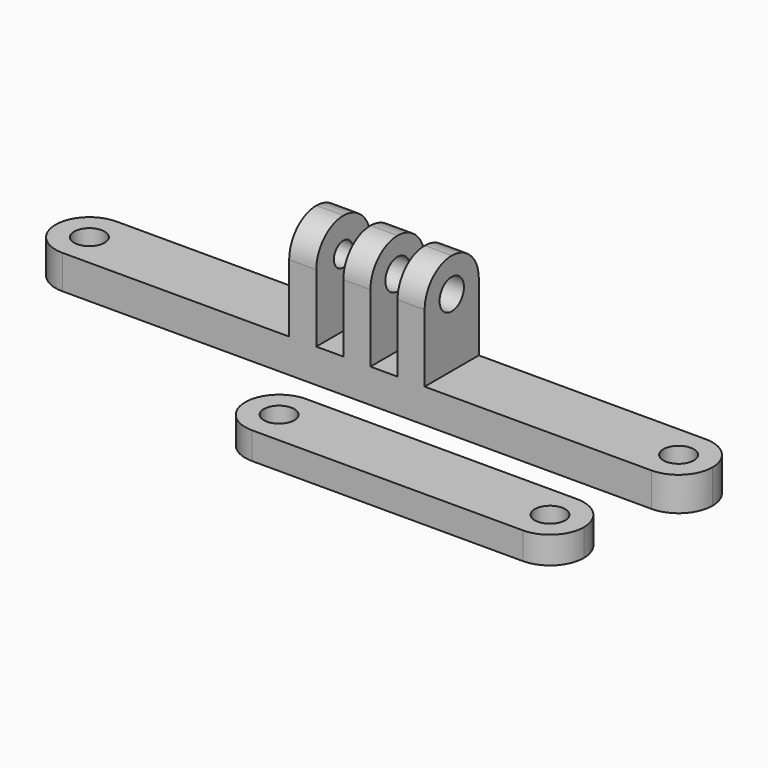
from build123d import *

# Parameters (mm, degrees)
F0_W     = 4
F0_H     = 15
F1_DEPTH = 5
F2_R     = 4.99999
F4_D     = 4.5
F6_D     = 4.5
F6_DEPTH = 50.501
F7_D     = 3.5
F9_DEPTH = 4
F10_D    = 4.5


# Not quite as in the source:
# - a fillet or chamfer is up to 0.001 mm smaller than in the source, because OpenCascade refuses the exact size


with BuildPart() as f1:
    # F0 (on Front) → F1 (new body, symmetric)
    with BuildSketch(Plane.XZ):
        with Locations((0, 12.5)):
            Rectangle(F0_W, F0_H)
        with Locations((8, 12.5)):
            Rectangle(F0_W, F0_H)
        with Locations((-8, 12.5)):
            Rectangle(F0_W, F0_H)
        Polygon((-48.5, 5), (-48.5, 0), (48.5, 0), (48.5, 5), (10, 5), (6, 5), (2, 5), (-2, 5), (-6, 5), (-10, 5), align=None)
    extrude(amount=F1_DEPTH, both=True)

    # F2 (radius 5 in the source; OpenCascade refuses exactly that, so slightly less here)
    f2_edges = [f1.edges().sort_by_distance(p)[0] for p in [
        (-48.5, -5, 2.5),
        (-48.5, 5, 2.5),
        (48.5, -5, 2.5),
        (48.5, 5, 2.5),
        (-8, -5, 20),
        (0, -5, 20),
        (8, -5, 20),
        (-8, 5, 20),
        (0, 5, 20),
        (8, 5, 20),
    ]]
    fillet(f2_edges, radius=F2_R)

    # F4 (through all)
    with Locations(Plane(origin=(0, 0, 0), x_dir=(1, 0, 0), z_dir=(0, 0, -1))):
        with Locations((-43.5, 0), (43.5, 0)):
            Hole(F4_D / 2)

    # F6 (through all, one way)
    with BuildSketch(Plane(origin=(-2, 0, 0), x_dir=(0, -1, 0), z_dir=(-1, 0, 0))):
        with Locations((0, 15)):
            Circle(F6_D / 2)
    extrude(amount=-F6_DEPTH, mode=Mode.SUBTRACT)

    # F7 (through all)
    with Locations(Plane(origin=(-2, 0, 0), x_dir=(0, -1, 0), z_dir=(1, 0, 0))):
        with Locations((0, -15)):
            Hole(F7_D / 2)


with BuildPart() as f9:
    # F8 (on Top) → F9 (new body)
    with BuildSketch(Plane.XY):
        with BuildLine():
            Line((40.0654178858, -14.444706738), (0.0654178858, -14.444706738))
            ThreePointArc((0.0654178858, -14.444706738), (-3.4701160202, -15.9091728321), (-4.9345821142, -19.444706738))
            ThreePointArc((-4.9345821142, -19.444706738), (-3.4701160202, -22.9802406439), (0.0654178858, -24.444706738))
            Line((0.0654178858, -24.444706738), (40.0654178858, -24.444706738))
            ThreePointArc((40.0654178858, -24.444706738), (43.6009517917, -22.9802406439), (45.0654178858, -19.444706738))
            ThreePointArc((45.0654178858, -19.444706738), (43.6009517917, -15.9091728321), (40.0654178858, -14.444706738))
        make_face()
    extrude(amount=F9_DEPTH)

    # F10 (through all)
    with Locations(Plane(origin=(0, 0, 0), x_dir=(1, 0, 0), z_dir=(0, 0, -1))):
        with Locations((0.0654178858, 19.444706738), (40.0654178858, 19.444706738)):
            Hole(F10_D / 2)


solid = Compound([f1.part, f9.part])
